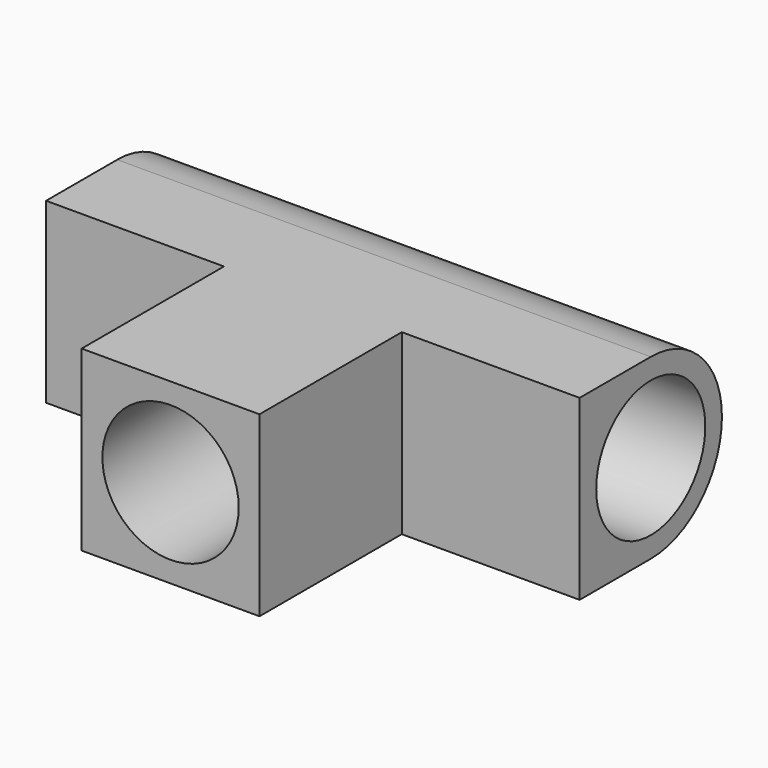
from build123d import *

# Parameters (mm, degrees)
F1_DEPTH = 30
F3_R     = 11.5
F4_DEPTH = 30
F2_R     = 11.5
F5_DEPTH = 90
F6_R     = 14.99999


# Not quite as in the source:
# - a fillet or chamfer is up to 0.001 mm smaller than in the source, because OpenCascade refuses the exact size


with BuildPart() as f1:
    # F0 (on Top) → F1 (new body)
    with BuildSketch(Plane.XY):
        Polygon((15, -15), (45, -15), (45, 15), (-45, 15), (-45, -15), (-15, -15), align=None)
        Polygon((15, -45), (15, -15), (-15, -15), (-15, -45), (0, -45), align=None)
    extrude(amount=F1_DEPTH)

    # F3 (on face) → F4 (cut)
    with BuildSketch(Plane.XZ.offset(45)):
        with Locations((0, 15)):
            Circle(F3_R)
    extrude(amount=-F4_DEPTH, mode=Mode.SUBTRACT)

    # F2 (on face) → F5 (cut)
    with BuildSketch(Plane(origin=(-45, 0, 0), x_dir=(0, -1, 0), z_dir=(-1, 0, 0))):
        with Locations((0, 15)):
            Circle(F2_R)
    extrude(amount=-F5_DEPTH, mode=Mode.SUBTRACT)

    # F6 (radius 15 in the source; OpenCascade refuses exactly that, so slightly less here)
    f6_edges = [f1.edges().sort_by_distance(p)[0] for p in [
        (0, 15, 0),
        (0, 15, 30),
    ]]
    fillet(f6_edges, radius=F6_R)


solid = f1.part
